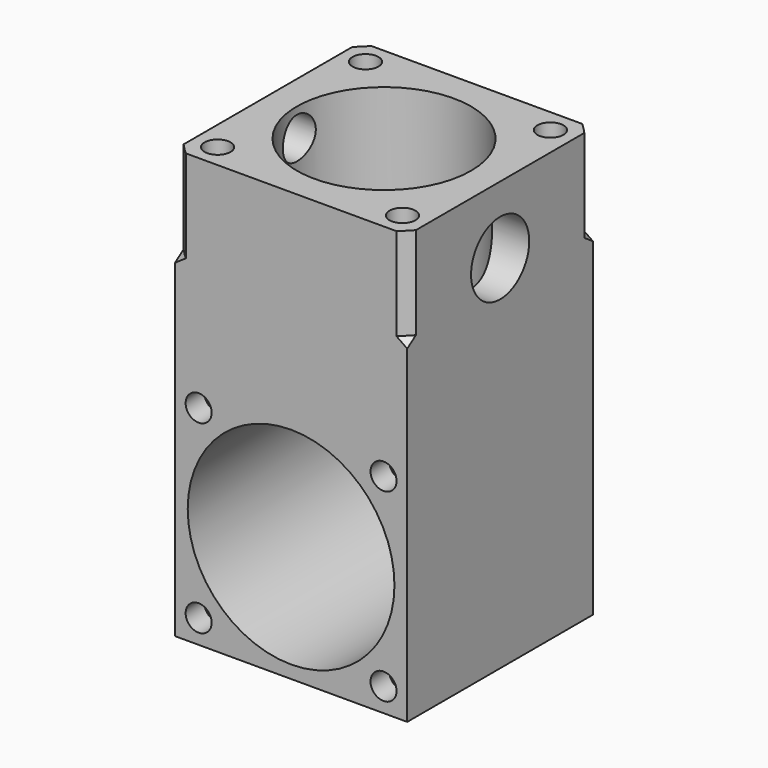
from build123d import *

# Parameters (mm, degrees)
F0_W         = 25.4
F0_H         = 25.4
F1_DEPTH     = 46.86
F3_DEPTH     = 11.11
F4_T4_ANGLE  = 22.8192997927
F4_T10_ANGLE = 22.8192997927
F4_T16_ANGLE = 22.8192997927
F4_T22_ANGLE = 22.8192997927
F5_R         = 2.2479
F6_DEPTH     = 6.4371526241
F8_R         = 9.525
F9_DEPTH     = 31.75
F10_R        = 1.4224
F11_DEPTH    = 7.9502
F7_R         = 11.303
F12_DEPTH    = 25.401
F7_R_2       = 1.4224
F13_DEPTH    = 2.5348692
F14_R        = 3.9751
F15_DEPTH    = 6.35
F16_R        = 1.4224
F17_DEPTH    = 5.715


# Not quite as in the source:
# - a fillet or chamfer that OpenCascade refuses, or shapes differently, is made with other operations: its cross-section is extruded or revolved along the edge and cut away or added


with BuildPart() as f1:
    # F0 (on Top) → F1 (new body)
    with BuildSketch(Plane.XY):
        Rectangle(F0_W, F0_H)
    extrude(amount=F1_DEPTH)

    # F2 (on face) → F3 (cut)
    with BuildSketch(Plane.XY.offset(46.86)):
        with BuildLine():
            ThreePointArc((-11.5104126772, -12.7), (-12.1198102295, -12.1198102295), (-12.7, -11.5104126772))
            Line((-12.7, -11.5104126772), (-12.7, -12.7))
            Line((-12.7, -12.7), (-11.5104126772, -12.7))
        make_face()
        with BuildLine():
            ThreePointArc((-12.7, 11.5104126772), (-12.1198102295, 12.1198102295), (-11.5104126772, 12.7))
            Line((-11.5104126772, 12.7), (-12.7, 12.7))
            Line((-12.7, 12.7), (-12.7, 11.5104126772))
        make_face()
        with BuildLine():
            Line((12.7, 12.7), (11.5104126772, 12.7))
            ThreePointArc((11.5104126772, 12.7), (12.1198102295, 12.1198102295), (12.7, 11.5104126772))
            Line((12.7, 11.5104126772), (12.7, 12.7))
        make_face()
        with BuildLine():
            Line((12.7, -12.7), (12.7, -11.5104126772))
            ThreePointArc((12.7, -11.5104126772), (12.1198102295, -12.1198102295), (11.5104126772, -12.7))
            Line((11.5104126772, -12.7), (12.7, -12.7))
        make_face()
    extrude(amount=-F3_DEPTH, mode=Mode.SUBTRACT)

    # F4: chamfer of 1 on 4 edges, made by hand


with BuildPart() as f4_tool2:
    # F4_s3 → F4_t4 (revolve)
    with BuildSketch(Plane(origin=(0, 0, 0), x_dir=(0, 0, 1), z_dir=(0.8330144325, -0.5532512587, 0))):
        Polygon((36.75, 17.14), (35.75, 18.14), (35.75, 17.14), align=None)
    revolve(axis=Axis((0, 0, 35.75), (0, 0, -1)), revolution_arc=F4_T4_ANGLE)

    split(bisect_by=Plane.XZ.offset(12.7), keep=Keep.BOTTOM)

    split(bisect_by=Plane.YZ.offset(-12.7), keep=Keep.TOP)


with BuildPart() as f1_1:
    add(f1.part)

    # F4_t1: union F4_tool2
    add(f4_tool2.part)


with BuildPart() as f4_tool8:
    # F4_s9 → F4_t10 (revolve)
    with BuildSketch(Plane(origin=(0, 0, 0), x_dir=(0, 0, 1), z_dir=(0.5532512587, 0.8330144325, 0))):
        Polygon((35.75, 18.14), (36.75, 17.14), (35.75, 17.14), align=None)
    revolve(axis=Axis((0, 0, 35.75), (0, 0, -1)), revolution_arc=F4_T10_ANGLE)

    split(bisect_by=Plane.XZ.offset(12.7), keep=Keep.BOTTOM)

    split(bisect_by=Plane.YZ.offset(12.7), keep=Keep.BOTTOM)


with BuildPart() as f1_2:
    add(f1_1.part)

    # F4_t7: union F4_tool8
    add(f4_tool8.part)


with BuildPart() as f4_tool14:
    # F4_s15 → F4_t16 (revolve)
    with BuildSketch(Plane(origin=(0, 0, 0), x_dir=(0, 0, 1), z_dir=(-0.8330144325, 0.5532512587, 0))):
        Polygon((35.75, 18.14), (36.75, 17.14), (35.75, 17.14), align=None)
    revolve(axis=Axis((0, 0, 35.75), (0, 0, -1)), revolution_arc=F4_T16_ANGLE)

    split(bisect_by=Plane.YZ.offset(12.7), keep=Keep.BOTTOM)

    split(bisect_by=Plane.XZ.offset(-12.7), keep=Keep.TOP)


with BuildPart() as f1_3:
    add(f1_2.part)

    # F4_t13: union F4_tool14
    add(f4_tool14.part)


with BuildPart() as f4_tool20:
    # F4_s21 → F4_t22 (revolve)
    with BuildSketch(Plane(origin=(0, 0, 0), x_dir=(0, 0, 1), z_dir=(-0.5532512587, -0.8330144325, 0))):
        Polygon((36.75, 17.14), (35.75, 18.14), (35.75, 17.14), align=None)
    revolve(axis=Axis((0, 0, 35.75), (0, 0, -1)), revolution_arc=F4_T22_ANGLE)

    split(bisect_by=Plane.YZ.offset(-12.7), keep=Keep.TOP)

    split(bisect_by=Plane.XZ.offset(-12.7), keep=Keep.TOP)


with BuildPart() as f1_4:
    add(f1_3.part)

    # F4_t19: union F4_tool20
    add(f4_tool20.part)

    # F5 (on face) → F6 (cut)
    with BuildSketch(Plane(origin=(-12.7, 0, 0), x_dir=(0, -1, 0), z_dir=(-1, 0, 0))):
        with Locations((0, 43.812)):
            Circle(F5_R)
    extrude(amount=-F6_DEPTH, mode=Mode.SUBTRACT)

    # F8 (on face) → F9 (cut)
    with BuildSketch(Plane.XY.offset(46.86)):
        Circle(F8_R)
    extrude(amount=-F9_DEPTH, mode=Mode.SUBTRACT)

    # F10 (on face) → F11 (cut)
    with BuildSketch(Plane.XY.offset(46.86)):
        with Locations((10.1092, -10.1092)):
            Circle(F10_R)
        with Locations((10.1092, 10.1092)):
            Circle(F10_R)
        with Locations((-10.1092, 10.1092)):
            Circle(F10_R)
        with Locations((-10.1092, -10.1092)):
            Circle(F10_R)
    extrude(amount=-F11_DEPTH, mode=Mode.SUBTRACT)

    # F7 (on face) → F12 (cut, through all)
    with BuildSketch(Plane.XZ.offset(12.7)):
        with Locations((0, 12.7)):
            Circle(F7_R)
    extrude(amount=-F12_DEPTH, mode=Mode.SUBTRACT)

    # F7 (on face) → F13 (cut)
    with BuildSketch(Plane.XZ.offset(12.7)):
        with Locations((10.1092, 22.8092)):
            Circle(F7_R_2)
        with Locations((10.1092, 2.5908)):
            Circle(F7_R_2)
        with Locations((-10.1092, 2.5908)):
            Circle(F7_R_2)
        with Locations((-10.1092, 22.8092)):
            Circle(F7_R_2)
    extrude(amount=-F13_DEPTH, mode=Mode.SUBTRACT)

    # F14 (on face) → F15 (cut)
    with BuildSketch(Plane.YZ.offset(12.7)):
        with Locations((0, 39.494)):
            Circle(F14_R)
    extrude(amount=-F15_DEPTH, mode=Mode.SUBTRACT)

    # F16 (on face) → F17 (cut)
    with BuildSketch(Plane(origin=(0, 12.7, 0), x_dir=(-1, 0, 0), z_dir=(0, 1, 0))):
        with Locations((-10.1092, 22.8092)):
            Circle(F16_R)
        with Locations((10.1092, 22.8092)):
            Circle(F16_R)
        with Locations((10.1092, 2.5908)):
            Circle(F16_R)
        with Locations((-10.1092, 2.5908)):
            Circle(F16_R)
    extrude(amount=-F17_DEPTH, mode=Mode.SUBTRACT)


solid = f1_4.part
